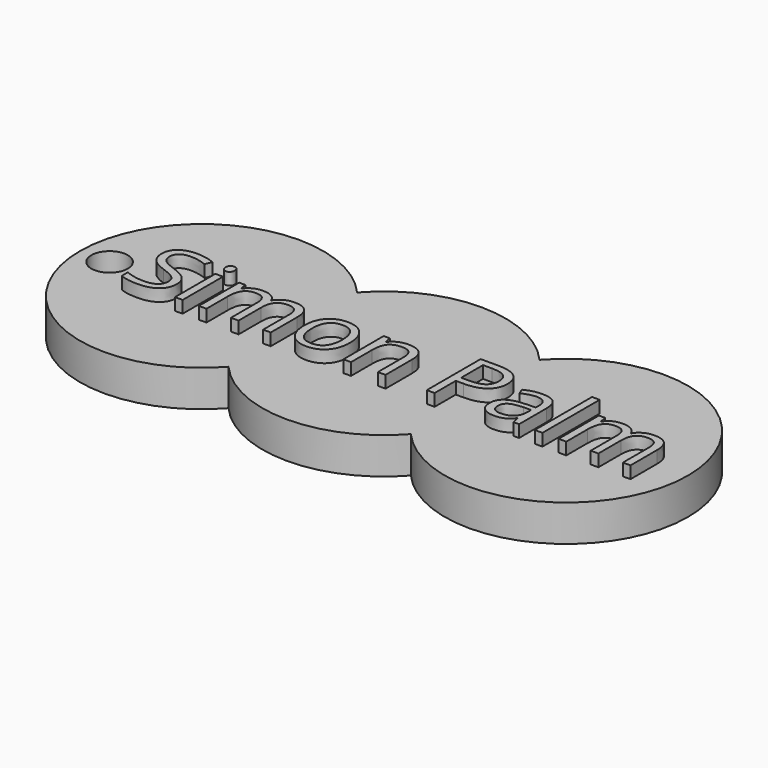
from build123d import *

# Parameters (mm, degrees)
F0_R         = 1.5
F1_DEPTH     = 3
F2_TEXT_SIZE = 7.747731676
F3_DEPTH     = 1


# Not quite as in the source:
# - Text() gives the source's letters only with a copy of the font that has no kerning and outlines rounded to 1/6400 em; it was checked with that copy


with BuildPart() as f1:
    # F0 (on Top) → F1 (new body)
    with BuildSketch(Plane.XY):
        with BuildLine():
            ThreePointArc((-7.5, 6.6143782777), (-25, 0), (-7.5, -6.6143782777))
            ThreePointArc((-7.5, -6.6143782777), (0, -10), (7.5, -6.6143782777))
            ThreePointArc((7.5, -6.6143782777), (25, 0), (7.5, 6.6143782777))
            ThreePointArc((7.5, 6.6143782777), (0, 10), (-7.5, 6.6143782777))
        make_face()
        with Locations((-22.5668940693, 0)):
            Circle(F0_R, mode=Mode.SUBTRACT)
    extrude(amount=F1_DEPTH)

    # F2 (on face) → F3 (join)
    with BuildSketch(Plane.XY.offset(3)):
        with Locations((-19.948144909, -2.6989260223)):
            Text('Simon Palm', F2_TEXT_SIZE, font='Open Sans', text_align=(TextAlign.LEFT, TextAlign.BOTTOM))
    extrude(amount=F3_DEPTH)


solid = f1.part
